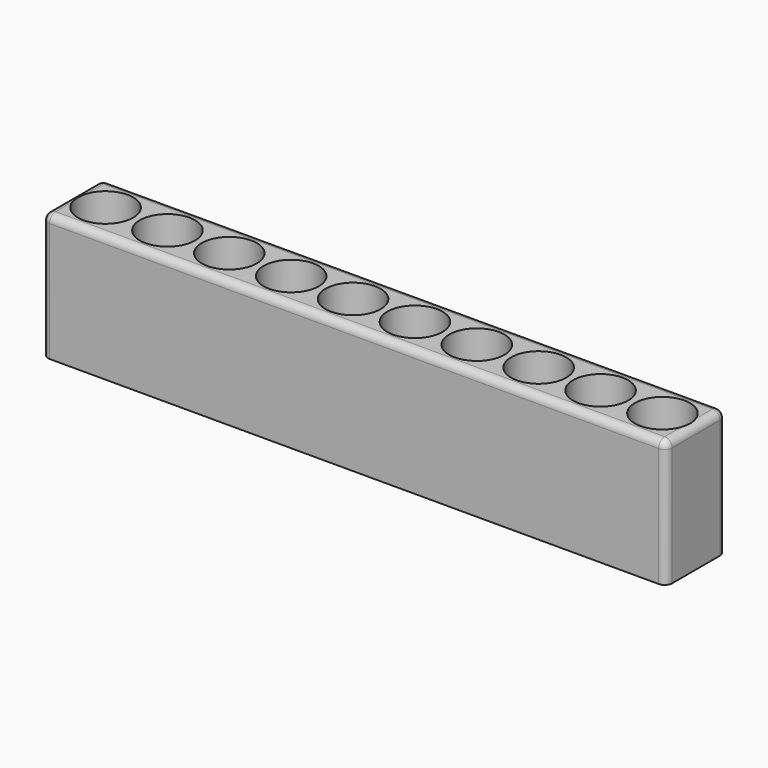
from build123d import *

# Parameters (mm, degrees)
F0_R         = 3.7
F1_DEPTH     = 17
F2_T1_DEPTH  = 81.7
F2_T3_DEPTH  = 8
F2_T6_ANGLE  = 90
F2_T8_ANGLE  = 90
F2_T10_ANGLE = 90
F2_T12_ANGLE = 90


# Not quite as in the source:
# - a fillet or chamfer that OpenCascade refuses, or shapes differently, is made with other operations: its cross-section is extruded or revolved along the edge and cut away or added


with BuildPart() as f1:
    # F0 (on Top) → F1 (new body)
    with BuildSketch(Plane.XY):
        with BuildLine():
            ThreePointArc((-4.5, -4), (-4.2071067812, -4.7071067812), (-3.5, -5))
            Line((-3.5, -5), (78.2, -5))
            ThreePointArc((78.2, -5), (78.9071067812, -4.7071067812), (79.2, -4))
            Line((79.2, -4), (79.2, 4))
            ThreePointArc((79.2, 4), (78.9071067812, 4.7071067812), (78.2, 5))
            Line((78.2, 5), (-3.5, 5))
            ThreePointArc((-3.5, 5), (-4.2071067812, 4.7071067812), (-4.5, 4))
            Line((-4.5, 4), (-4.5, -4))
        make_face()
        Circle(F0_R, mode=Mode.SUBTRACT)
        with Locations((8.3, 0)):
            Circle(F0_R, mode=Mode.SUBTRACT)
        with Locations((16.6, 0)):
            Circle(F0_R, mode=Mode.SUBTRACT)
        with Locations((24.9, 0)):
            Circle(F0_R, mode=Mode.SUBTRACT)
        with Locations((33.2, 0)):
            Circle(F0_R, mode=Mode.SUBTRACT)
        with Locations((41.5, 0)):
            Circle(F0_R, mode=Mode.SUBTRACT)
        with Locations((49.8, 0)):
            Circle(F0_R, mode=Mode.SUBTRACT)
        with Locations((58.1, 0)):
            Circle(F0_R, mode=Mode.SUBTRACT)
        with Locations((66.4, 0)):
            Circle(F0_R, mode=Mode.SUBTRACT)
        with Locations((74.7, 0)):
            Circle(F0_R, mode=Mode.SUBTRACT)
    extrude(amount=F1_DEPTH)

    # F2: fillet of radius 1 on 8 edges, made by hand

    # F2_s2 → F2_t1 (cut)
    with BuildSketch(Plane.YZ.offset(-3.5)):
        with BuildLine():
            ThreePointArc((-5, 16), (-4.7071067812, 16.7071067812), (-4, 17))
            Line((-4, 17), (-5, 17))
            Line((-5, 17), (-5, 16))
        make_face()
        with BuildLine():
            ThreePointArc((5, 16), (4.7071067812, 16.7071067812), (4, 17))
            Line((4, 17), (5, 17))
            Line((5, 17), (5, 16))
        make_face()
    extrude(amount=F2_T1_DEPTH, mode=Mode.SUBTRACT)

    # F2_s4 → F2_t3 (cut)
    with BuildSketch(Plane.XZ.offset(-4)):
        with BuildLine():
            ThreePointArc((79.2, 16), (78.9071067812, 16.7071067812), (78.2, 17))
            Line((78.2, 17), (79.2, 17))
            Line((79.2, 17), (79.2, 16))
        make_face()
        with BuildLine():
            ThreePointArc((-4.5, 16), (-4.2071067812, 16.7071067812), (-3.5, 17))
            Line((-3.5, 17), (-4.5, 17))
            Line((-4.5, 17), (-4.5, 16))
        make_face()
    extrude(amount=F2_T3_DEPTH, mode=Mode.SUBTRACT)

    # F2_s5 → F2_t6 (revolve, cut)
    with BuildSketch(Plane.XZ.offset(4)):
        with BuildLine():
            ThreePointArc((-4.5, 16), (-4.2071067812, 16.7071067812), (-3.5, 17))
            Line((-3.5, 17), (-4.5, 17))
            Line((-4.5, 17), (-4.5, 16))
        make_face()
    revolve(axis=Axis((-3.5, -4, 17), (0, 0, 1)), revolution_arc=F2_T6_ANGLE, mode=Mode.SUBTRACT)

    # F2_s7 → F2_t8 (revolve, cut)
    with BuildSketch(Plane.YZ.offset(78.2)):
        with BuildLine():
            ThreePointArc((-5, 16), (-4.7071067812, 16.7071067812), (-4, 17))
            Line((-4, 17), (-5, 17))
            Line((-5, 17), (-5, 16))
        make_face()
    revolve(axis=Axis((78.2, -4, 17), (0, 0, 1)), revolution_arc=F2_T8_ANGLE, mode=Mode.SUBTRACT)

    # F2_s9 → F2_t10 (revolve, cut)
    with BuildSketch(Plane.XZ.offset(-4)):
        with BuildLine():
            ThreePointArc((79.2, 16), (78.9071067812, 16.7071067812), (78.2, 17))
            Line((78.2, 17), (79.2, 17))
            Line((79.2, 17), (79.2, 16))
        make_face()
    revolve(axis=Axis((78.2, 4, 17), (0, 0, 1)), revolution_arc=F2_T10_ANGLE, mode=Mode.SUBTRACT)

    # F2_s11 → F2_t12 (revolve, cut)
    with BuildSketch(Plane.YZ.offset(-3.5)):
        with BuildLine():
            ThreePointArc((5, 16), (4.7071067812, 16.7071067812), (4, 17))
            Line((4, 17), (5, 17))
            Line((5, 17), (5, 16))
        make_face()
    revolve(axis=Axis((-3.5, 4, 17), (0, 0, 1)), revolution_arc=F2_T12_ANGLE, mode=Mode.SUBTRACT)


solid = f1.part
